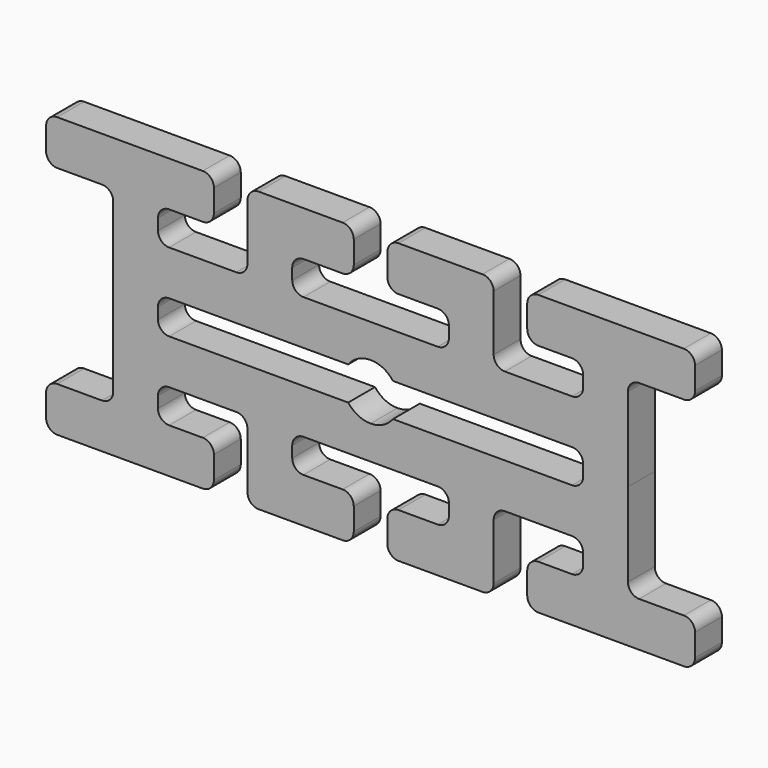
from build123d import *

# Parameters (mm, degrees)
F1_DEPTH = 3


# Not quite as in the source:
# - a feature names something its author has since deleted; it is built from what else it names


with BuildPart() as f1:
    # F0 (on Front) → F1 (new body)
    with BuildSketch(Plane.XZ):
        with BuildLine():
            Line((-23.0000003952, 0), (-19.0015753579, 0))
            Line((-19.0015753579, 0), (-19.0015753579, 0.5))
            ThreePointArc((-19.0015753579, 0.5), (-18.7086821391, 1.2071067812), (-18.0015753579, 1.5))
            Line((-18.0015753579, 1.5), (-2, 1.5))
            ThreePointArc((-2, 1.5), (-1.1180339887, 2.2360679775), (0, 2.5))
            Line((0, 2.5), (0, 5.4957361976))
            Line((0, 5.4957361976), (-6.0015753579, 5.4957361976))
            ThreePointArc((-6.0015753579, 5.4957361976), (-6.7086821391, 5.7886294164), (-7.0015753579, 6.4957361976))
            Line((-7.0015753579, 6.4957361976), (-7.0015753579, 7.4957361976))
            ThreePointArc((-7.0015753579, 7.4957361976), (-6.7086821391, 8.2028429788), (-6.0015753579, 8.4957361976))
            Line((-6.0015753579, 8.4957361976), (-2.5015753579, 8.4957361976))
            ThreePointArc((-2.5015753579, 8.4957361976), (-1.7944685767, 8.7886294164), (-1.5015753579, 9.4957361976))
            Line((-1.5015753579, 9.4957361976), (-1.5015753579, 11.4957361976))
            ThreePointArc((-1.5015753579, 11.4957361976), (-1.7944685767, 12.2028429788), (-2.5015753579, 12.4957361976))
            Line((-2.5015753579, 12.4957361976), (-10.0015753579, 12.4957361976))
            ThreePointArc((-10.0015753579, 12.4957361976), (-10.7086821391, 12.2028429788), (-11.0015753579, 11.4957361976))
            Line((-11.0015753579, 11.4957361976), (-11.0015753579, 8.4957361976))
            Line((-11.0015753579, 8.4957361976), (-11.0015753579, 6.4957361976))
            ThreePointArc((-11.0015753579, 6.4957361976), (-11.2944685767, 5.7886294164), (-12.0015753579, 5.4957361976))
            Line((-12.0015753579, 5.4957361976), (-18.0015753579, 5.4957361976))
            ThreePointArc((-18.0015753579, 5.4957361976), (-18.7086821391, 5.7886294164), (-19.0015753579, 6.4957361976))
            Line((-19.0015753579, 6.4957361976), (-19.0015753579, 7.4957361976))
            ThreePointArc((-19.0015753579, 7.4957361976), (-18.7086821391, 8.2028429788), (-18.0015753579, 8.4957361976))
            Line((-18.0015753579, 8.4957361976), (-15.0015753579, 8.4957361976))
            ThreePointArc((-15.0015753579, 8.4957361976), (-14.2944685767, 8.7886294164), (-14.0015753579, 9.4957361976))
            Line((-14.0015753579, 9.4957361976), (-14.0015753579, 11.4957361976))
            ThreePointArc((-14.0015753579, 11.4957361976), (-14.2944685767, 12.2028429788), (-15.0015753579, 12.4957361976))
            Line((-15.0015753579, 12.4957361976), (-28.0015753579, 12.4957361976))
            ThreePointArc((-28.0015753579, 12.4957361976), (-28.7086821391, 12.2028429788), (-29.0015753579, 11.4957361976))
            Line((-29.0015753579, 11.4957361976), (-29.0015753579, 9.4957361976))
            ThreePointArc((-29.0015753579, 9.4957361976), (-28.7086821391, 8.7886294164), (-28.0015753579, 8.4957361976))
            Line((-28.0015753579, 8.4957361976), (-24.0015753579, 8.4957361976))
            ThreePointArc((-24.0015753579, 8.4957361976), (-23.294403037, 8.2028542282), (-23.0013899752, 7.4957362148))
            Line((-23.0013899752, 7.4957362148), (-23.0000003952, 0))
        make_face()
        with BuildLine():
            Line((19.0015753579, 0.5), (19.0015753579, 0))
            Line((19.0015753579, 0), (23.0000003952, 0))
            Line((23.0000003952, 0), (23.0013899752, 7.4957362148))
            ThreePointArc((23.0013899752, 7.4957362148), (23.294403037, 8.2028542282), (24.0015753579, 8.4957361976))
            Line((24.0015753579, 8.4957361976), (28.0015753579, 8.4957361976))
            ThreePointArc((28.0015753579, 8.4957361976), (28.7086821391, 8.7886294164), (29.0015753579, 9.4957361976))
            Line((29.0015753579, 9.4957361976), (29.0015753579, 11.4957361976))
            ThreePointArc((29.0015753579, 11.4957361976), (28.7086821391, 12.2028429788), (28.0015753579, 12.4957361976))
            Line((28.0015753579, 12.4957361976), (15.0015753579, 12.4957361976))
            ThreePointArc((15.0015753579, 12.4957361976), (14.2944685767, 12.2028429788), (14.0015753579, 11.4957361976))
            Line((14.0015753579, 11.4957361976), (14.0015753579, 9.4957361976))
            ThreePointArc((14.0015753579, 9.4957361976), (14.2944685767, 8.7886294164), (15.0015753579, 8.4957361976))
            Line((15.0015753579, 8.4957361976), (18.0015753579, 8.4957361976))
            ThreePointArc((18.0015753579, 8.4957361976), (18.7086821391, 8.2028429788), (19.0015753579, 7.4957361976))
            Line((19.0015753579, 7.4957361976), (19.0015753579, 6.4957361976))
            ThreePointArc((19.0015753579, 6.4957361976), (18.7086821391, 5.7886294164), (18.0015753579, 5.4957361976))
            Line((18.0015753579, 5.4957361976), (12.0015753579, 5.4957361976))
            ThreePointArc((12.0015753579, 5.4957361976), (11.2944685767, 5.7886294164), (11.0015753579, 6.4957361976))
            Line((11.0015753579, 6.4957361976), (11.0015753579, 8.4957361976))
            Line((11.0015753579, 8.4957361976), (11.0015753579, 11.4957361976))
            ThreePointArc((11.0015753579, 11.4957361976), (10.7086821391, 12.2028429788), (10.0015753579, 12.4957361976))
            Line((10.0015753579, 12.4957361976), (2.5015753579, 12.4957361976))
            ThreePointArc((2.5015753579, 12.4957361976), (1.7944685767, 12.2028429788), (1.5015753579, 11.4957361976))
            Line((1.5015753579, 11.4957361976), (1.5015753579, 9.4957361976))
            ThreePointArc((1.5015753579, 9.4957361976), (1.7944685767, 8.7886294164), (2.5015753579, 8.4957361976))
            Line((2.5015753579, 8.4957361976), (6.0015753579, 8.4957361976))
            ThreePointArc((6.0015753579, 8.4957361976), (6.7086821391, 8.2028429788), (7.0015753579, 7.4957361976))
            Line((7.0015753579, 7.4957361976), (7.0015753579, 6.4957361976))
            ThreePointArc((7.0015753579, 6.4957361976), (6.7086821391, 5.7886294164), (6.0015753579, 5.4957361976))
            Line((6.0015753579, 5.4957361976), (0, 5.4957361976))
            Line((0, 5.4957361976), (0, 2.5))
            ThreePointArc((0, 2.5), (1.1180339887, 2.2360679775), (2, 1.5))
            Line((2, 1.5), (18.0015753579, 1.5))
            ThreePointArc((18.0015753579, 1.5), (18.7086821391, 1.2071067812), (19.0015753579, 0.5))
        make_face()
        with BuildLine():
            Line((-6.0015753579, -5.4957361976), (0, -5.4957361976))
            Line((0, -5.4957361976), (0, -2.5))
            ThreePointArc((0, -2.5), (-1.1180339887, -2.2360679775), (-2, -1.5))
            Line((-2, -1.5), (-18.0015753579, -1.5))
            ThreePointArc((-18.0015753579, -1.5), (-18.7086821391, -1.2071067812), (-19.0015753579, -0.5))
            Line((-19.0015753579, -0.5), (-19.0015753579, 0))
            Line((-19.0015753579, 0), (-23.0000003952, 0))
            Line((-23.0000003952, 0), (-23.0013899752, -7.4957362148))
            ThreePointArc((-23.0013899752, -7.4957362148), (-23.294403037, -8.2028542282), (-24.0015753579, -8.4957361976))
            Line((-24.0015753579, -8.4957361976), (-28.0015753579, -8.4957361976))
            ThreePointArc((-28.0015753579, -8.4957361976), (-28.7086821391, -8.7886294164), (-29.0015753579, -9.4957361976))
            Line((-29.0015753579, -9.4957361976), (-29.0015753579, -11.4957361976))
            ThreePointArc((-29.0015753579, -11.4957361976), (-28.7086821391, -12.2028429788), (-28.0015753579, -12.4957361976))
            Line((-28.0015753579, -12.4957361976), (-15.0015753579, -12.4957361976))
            ThreePointArc((-15.0015753579, -12.4957361976), (-14.2944685767, -12.2028429788), (-14.0015753579, -11.4957361976))
            Line((-14.0015753579, -11.4957361976), (-14.0015753579, -9.4957361976))
            ThreePointArc((-14.0015753579, -9.4957361976), (-14.2944685767, -8.7886294164), (-15.0015753579, -8.4957361976))
            Line((-15.0015753579, -8.4957361976), (-18.0015753579, -8.4957361976))
            ThreePointArc((-18.0015753579, -8.4957361976), (-18.7086821391, -8.2028429788), (-19.0015753579, -7.4957361976))
            Line((-19.0015753579, -7.4957361976), (-19.0015753579, -6.4957361976))
            ThreePointArc((-19.0015753579, -6.4957361976), (-18.7086821391, -5.7886294164), (-18.0015753579, -5.4957361976))
            Line((-18.0015753579, -5.4957361976), (-12.0015753579, -5.4957361976))
            ThreePointArc((-12.0015753579, -5.4957361976), (-11.2944685767, -5.7886294164), (-11.0015753579, -6.4957361976))
            Line((-11.0015753579, -6.4957361976), (-11.0015753579, -8.4957361976))
            Line((-11.0015753579, -8.4957361976), (-11.0015753579, -11.4957361976))
            ThreePointArc((-11.0015753579, -11.4957361976), (-10.7086821391, -12.2028429788), (-10.0015753579, -12.4957361976))
            Line((-10.0015753579, -12.4957361976), (-2.5015753579, -12.4957361976))
            ThreePointArc((-2.5015753579, -12.4957361976), (-1.7944685767, -12.2028429788), (-1.5015753579, -11.4957361976))
            Line((-1.5015753579, -11.4957361976), (-1.5015753579, -9.4957361976))
            ThreePointArc((-1.5015753579, -9.4957361976), (-1.7944685767, -8.7886294164), (-2.5015753579, -8.4957361976))
            Line((-2.5015753579, -8.4957361976), (-6.0015753579, -8.4957361976))
            ThreePointArc((-6.0015753579, -8.4957361976), (-6.7086821391, -8.2028429788), (-7.0015753579, -7.4957361976))
            Line((-7.0015753579, -7.4957361976), (-7.0015753579, -6.4957361976))
            ThreePointArc((-7.0015753579, -6.4957361976), (-6.7086821391, -5.7886294164), (-6.0015753579, -5.4957361976))
        make_face()
        with BuildLine():
            ThreePointArc((1.5015753579, -11.4957361976), (1.7944685767, -12.2028429788), (2.5015753579, -12.4957361976))
            Line((2.5015753579, -12.4957361976), (10.0015753579, -12.4957361976))
            ThreePointArc((10.0015753579, -12.4957361976), (10.7086821391, -12.2028429788), (11.0015753579, -11.4957361976))
            Line((11.0015753579, -11.4957361976), (11.0015753579, -8.4957361976))
            Line((11.0015753579, -8.4957361976), (11.0015753579, -6.4957361976))
            ThreePointArc((11.0015753579, -6.4957361976), (11.2944685767, -5.7886294164), (12.0015753579, -5.4957361976))
            Line((12.0015753579, -5.4957361976), (18.0015753579, -5.4957361976))
            ThreePointArc((18.0015753579, -5.4957361976), (18.7086821391, -5.7886294164), (19.0015753579, -6.4957361976))
            Line((19.0015753579, -6.4957361976), (19.0015753579, -7.4957361976))
            ThreePointArc((19.0015753579, -7.4957361976), (18.7086821391, -8.2028429788), (18.0015753579, -8.4957361976))
            Line((18.0015753579, -8.4957361976), (15.0015753579, -8.4957361976))
            ThreePointArc((15.0015753579, -8.4957361976), (14.2944685767, -8.7886294164), (14.0015753579, -9.4957361976))
            Line((14.0015753579, -9.4957361976), (14.0015753579, -11.4957361976))
            ThreePointArc((14.0015753579, -11.4957361976), (14.2944685767, -12.2028429788), (15.0015753579, -12.4957361976))
            Line((15.0015753579, -12.4957361976), (28.0015753579, -12.4957361976))
            ThreePointArc((28.0015753579, -12.4957361976), (28.7086821391, -12.2028429788), (29.0015753579, -11.4957361976))
            Line((29.0015753579, -11.4957361976), (29.0015753579, -9.4957361976))
            ThreePointArc((29.0015753579, -9.4957361976), (28.7086821391, -8.7886294164), (28.0015753579, -8.4957361976))
            Line((28.0015753579, -8.4957361976), (24.0015753579, -8.4957361976))
            ThreePointArc((24.0015753579, -8.4957361976), (23.294403037, -8.2028542282), (23.0013899752, -7.4957362148))
            Line((23.0013899752, -7.4957362148), (23.0000003952, 0))
            Line((23.0000003952, 0), (19.0015753579, 0))
            Line((19.0015753579, 0), (19.0015753579, -0.5))
            ThreePointArc((19.0015753579, -0.5), (18.7086821391, -1.2071067812), (18.0015753579, -1.5))
            Line((18.0015753579, -1.5), (2, -1.5))
            ThreePointArc((2, -1.5), (1.1180339887, -2.2360679775), (0, -2.5))
            Line((0, -2.5), (0, -5.4957361976))
            Line((0, -5.4957361976), (6.0015753579, -5.4957361976))
            ThreePointArc((6.0015753579, -5.4957361976), (6.7086821391, -5.7886294164), (7.0015753579, -6.4957361976))
            Line((7.0015753579, -6.4957361976), (7.0015753579, -7.4957361976))
            ThreePointArc((7.0015753579, -7.4957361976), (6.7086821391, -8.2028429788), (6.0015753579, -8.4957361976))
            Line((6.0015753579, -8.4957361976), (2.5015753579, -8.4957361976))
            ThreePointArc((2.5015753579, -8.4957361976), (1.7944685767, -8.7886294164), (1.5015753579, -9.4957361976))
            Line((1.5015753579, -9.4957361976), (1.5015753579, -11.4957361976))
        make_face()
    extrude(amount=F1_DEPTH)


solid = f1.part
